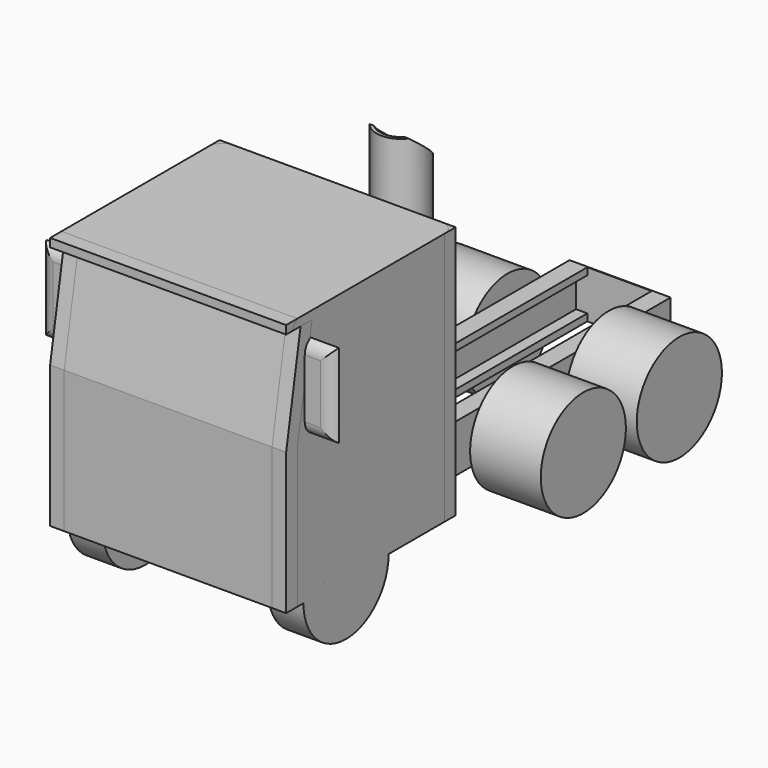
from build123d import *

# Parameters (mm, degrees)
F0_W          = 84.9026963115
F0_H          = 91.2344232202
F1_DEPTH      = 38.1
F3_DEPTH      = 42.4523481557
F3_DEPTH_BACK = 42.4523481557
F4_R          = 19.1453288311
F5_DEPTH      = 12.7
F8_DEPTH      = 127
F10_R         = 19.1453262
F11_DEPTH     = 25.4
F13_R         = 5.08
F14_T1_DEPTH  = 111.0309954692
F15_R         = 8.8626036941
F16_DEPTH     = 101.6
F17_R         = 7.6745278719
F18_DEPTH     = 99.06
F20_DEPTH     = 43.5794721032
F21_W         = 2.6513483719
F21_H         = 30.1193892955
F22_DEPTH     = 10.16
F23_T1_DEPTH  = 32.4692196578
F23_T3_DEPTH  = 52.4286089533
F26_DEPTH     = 0.254


# Not quite as in the source:
# - a fillet or chamfer that OpenCascade refuses, or shapes differently, is made with other operations: its cross-section is extruded or revolved along the edge and cut away or added


with BuildPart() as f1:
    # F0 (on Front) → F1 (new body, symmetric)
    with BuildSketch(Plane.XZ):
        Rectangle(F0_W, F0_H)
    extrude(amount=F1_DEPTH, both=True)

    # F2 (on Right) → F3 (cut, two sides)
    with BuildSketch(Plane.YZ) as f3_sk:
        Polygon((-38.9483012259, 42.5993576646), (-38.1342619658, 5.1536280662), (-31.6219590604, 42.5993576646), align=None)
    extrude(amount=-F3_DEPTH, mode=Mode.SUBTRACT)
    extrude(f3_sk.sketch, amount=F3_DEPTH_BACK, mode=Mode.SUBTRACT)

    # F4 (on face) → F5 (join)
    with BuildSketch(Plane.YZ.offset(42.4513481557)):
        with Locations((-11.1792916432, -45.6172116101)):
            Circle(F4_R)
    extrude(amount=-F5_DEPTH)


with BuildPart() as f6_1:
    # F6: instance of F1
    add(f1.part.mirror(Plane.YZ))


with BuildPart() as f8:
    # F7 (on face) → F8 (new body)
    with BuildSketch(Plane(origin=(0, 38.1, 0), x_dir=(-1, 0, 0), z_dir=(0, 1, 0))):
        Polygon((-18.1784721032, -53.2778071603), (-11.5744721032, -53.2778071603), (-11.5744721032, -50.7378071603), (-15.6384721032, -50.7378071603), (-15.6384721032, -38.6785142068), (-11.5744721032, -38.6785142068), (-11.5744721032, -36.1385142068), (-18.1784721032, -36.1385142068), align=None)
    extrude(amount=F8_DEPTH)


with BuildPart() as f9_1:
    # F9: instance of F8
    add(f8.part.mirror(Plane.YZ))


with BuildPart() as f8_1:
    add(f8.part)

    # F10 (on face) → F11 (join)
    with BuildSketch(Plane.YZ.offset(18.1784721032)):
        with Locations((137.2673511505, -48.1978071603)):
            Circle(F10_R)
        with Locations((94.0964892507, -48.1978071603)):
            Circle(F10_R)
    extrude(amount=F11_DEPTH)


with BuildPart() as f12_1:
    # F12: instance of F8
    add(f8_1.part.mirror(Plane.YZ))


with BuildPart() as f1_1:
    add(f1.part)

    # F13
    f13_edges = [f1_1.edges().sort_by_distance(p)[0] for p in [
        (42.451348, -38.1, -20.133289),
        (42.451348, -34.86098, 23.974996),
        (-42.451348, -38.1, -20.133289),
        (-42.451348, -34.86098, 23.974996),
        (42.451348, 38.1, 0),
        (-42.451348, 38.1, 0),
    ]]
    fillet(f13_edges, radius=F13_R)

    # F14: chamfer of 5.08 on 1 edges, made by hand

    # F14_s2 → F14_t1 (cut)
    with BuildSketch(Plane.YZ.offset(-55.5154977346)):
        Polygon((-33.02, 45.6172116101), (-38.1, 40.5372116101), (-38.1, 45.6172116101), align=None)
    extrude(amount=F14_T1_DEPTH, mode=Mode.SUBTRACT)


with BuildPart() as f8_2:
    add(f8_1.part)

    # F15 (on face) → F16 (join)
    with BuildSketch(Plane.XY.offset(-36.1385142068)):
        with Locations((15.265696682, 47.6398468018)):
            Circle(F15_R)
    extrude(amount=F16_DEPTH)

    # F17 (on face) → F18 (cut)
    with BuildSketch(Plane.XY.offset(65.4614857932)):
        with Locations((15.265696682, 47.6398468018)):
            Circle(F17_R)
    extrude(amount=-F18_DEPTH, mode=Mode.SUBTRACT)

    # F19 (on Right) → F20 (cut, through all)
    with BuildSketch(Plane.YZ):
        Polygon((58.7693750858, 70.7835555077), (33.8418483734, 72.4776536226), (58.7693750858, 51.6643822193), align=None)
    extrude(amount=F20_DEPTH, mode=Mode.SUBTRACT)


with BuildPart() as f22:
    # F21 (on face) → F22 (new body)
    with BuildSketch(Plane.YZ.offset(42.4513481557)):
        with Locations((-28.417179361, 22.1676826477)):
            Rectangle(F21_W, F21_H)
    extrude(amount=F22_DEPTH)

    # F23: fillet of radius 5.08 on 3 edges, made by hand

    # F23_s2 → F23_t1 (cut)
    with BuildSketch(Plane.YZ.offset(31.2967383268)):
        with BuildLine():
            ThreePointArc((-27.091505175, 37.2273772955), (-29.0300008006, 35.360610408), (-29.742853547, 32.7655333639))
            Line((-29.742853547, 32.7655333639), (-29.742853547, 37.2273772955))
            Line((-29.742853547, 37.2273772955), (-27.091505175, 37.2273772955))
        make_face()
        with BuildLine():
            ThreePointArc((-29.742853547, 11.5698319316), (-29.0300008006, 8.9747548875), (-27.091505175, 7.107988))
            Line((-27.091505175, 7.107988), (-29.742853547, 7.107988))
            Line((-29.742853547, 7.107988), (-29.742853547, 11.5698319316))
        make_face()
    extrude(amount=F23_T1_DEPTH, mode=Mode.SUBTRACT)

    # F23_s4 → F23_t3 (cut)
    with BuildSketch(Plane.XY.offset(-4.0466218289)):
        with BuildLine():
            ThreePointArc((48.1495042242, -29.742853547), (50.7445812683, -29.0300008006), (52.6113481557, -27.091505175))
            Line((52.6113481557, -27.091505175), (52.6113481557, -29.742853547))
            Line((52.6113481557, -29.742853547), (48.1495042242, -29.742853547))
        make_face()
    extrude(amount=F23_T3_DEPTH, mode=Mode.SUBTRACT)


with BuildPart() as f24_1:
    # F24: instance of F22
    add(f22.part.mirror(Plane.YZ))


with BuildPart() as f26:
    # F25 (on face) → F26 (new body)
    with BuildSketch(Plane(origin=(0, 165.1, 0), x_dir=(-1, 0, 0), z_dir=(0, 1, 0))):
        Polygon((18.1113947183, -53.2778071603), (18.1086789817, -36.1547134817), (-18.1784721032, -36.1385142068), (-18.1784721032, -53.2778071603), align=None)
    extrude(amount=-F26_DEPTH)


solid = Compound([f6_1.part, f9_1.part, f12_1.part, f1_1.part, f8_2.part, f22.part, f24_1.part, f26.part])
